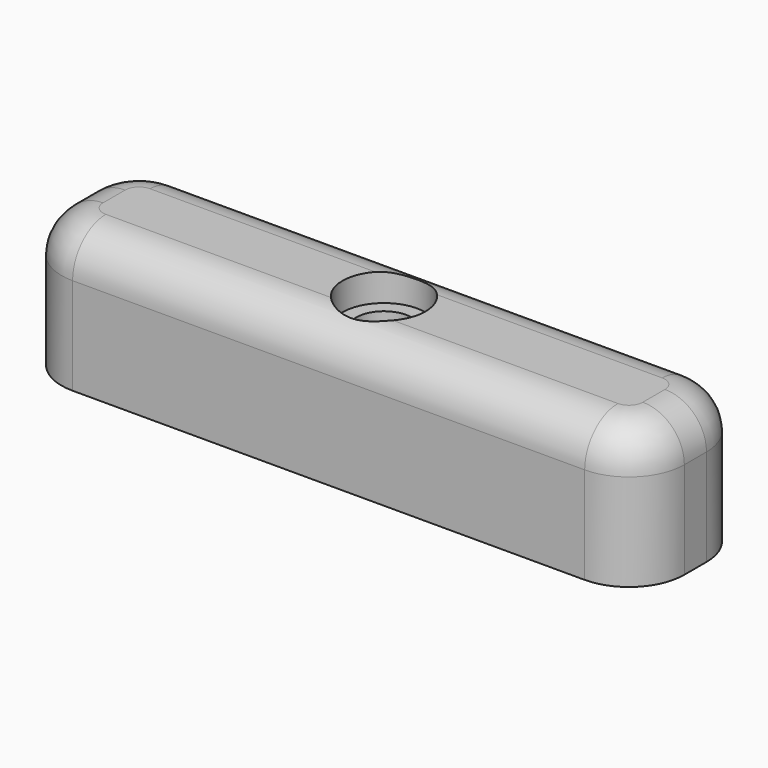
from build123d import *

# Parameters (mm, degrees)
F0_W     = 45
F0_H     = 10
F0_R     = 3
F0_R_2   = 2
F1_DEPTH = 10
F2_R     = 4
F3_R     = 3
F5_DEPTH = 2


with BuildPart() as f1:
    # F0 (on Top) → F1 (new body)
    with BuildSketch(Plane.XY):
        Rectangle(F0_W, F0_H)
        Circle(F0_R, mode=Mode.SUBTRACT)
        Circle(F0_R)
        Circle(F0_R_2, mode=Mode.SUBTRACT)
    extrude(amount=F1_DEPTH)

    # F2
    f2_edges = [f1.edges().sort_by_distance(p)[0] for p in [
        (-22.5, -5, 5),
        (22.5, -5, 5),
        (22.5, 5, 5),
        (-22.5, 5, 5),
    ]]
    fillet(f2_edges, radius=F2_R)

    # F3
    f3_edges = [f1.edges().sort_by_distance(p)[0] for p in [
        (0, -5, 10),
        (0, 5, 10),
        (21.328427, 3.828427, 10),
        (-21.328427, 3.828427, 10),
        (22.5, 0, 10),
        (-22.5, 0, 10),
        (21.328427, -3.828427, 10),
        (-21.328427, -3.828427, 10),
    ]]
    fillet(f3_edges, radius=F3_R)

    # F4 (on face) → F5 (cut)
    with BuildSketch(Plane.XY.offset(10)):
        with BuildLine():
            ThreePointArc((0, 2), (1.4142135624, 1.4142135624), (2, 0))
            ThreePointArc((2, 0), (1.4142135624, -1.4142135624), (0, -2))
            Line((0, -2), (2.2360679775, -2))
            ThreePointArc((2.2360679775, -2), (2.8025170769, -1.0704662693), (3, 0))
            ThreePointArc((3, 0), (2.8025170769, 1.0704662693), (2.2360679775, 2))
            Line((2.2360679775, 2), (0, 2))
        make_face()
        with BuildLine():
            Line((-2.2360679775, 2), (0, 2))
            Line((0, 2), (2.2360679775, 2))
            ThreePointArc((2.2360679775, 2), (0, 3), (-2.2360679775, 2))
        make_face()
        with BuildLine():
            ThreePointArc((0, -2), (-2, 0), (0, 2))
            Line((0, 2), (-2.2360679775, 2))
            ThreePointArc((-2.2360679775, 2), (-3, 0), (-2.2360679775, -2))
            Line((-2.2360679775, -2), (0, -2))
        make_face()
        with BuildLine():
            Line((2.2360679775, -2), (0, -2))
            Line((0, -2), (-2.2360679775, -2))
            ThreePointArc((-2.2360679775, -2), (0, -3), (2.2360679775, -2))
        make_face()
    extrude(amount=-F5_DEPTH, mode=Mode.SUBTRACT)


solid = f1.part
